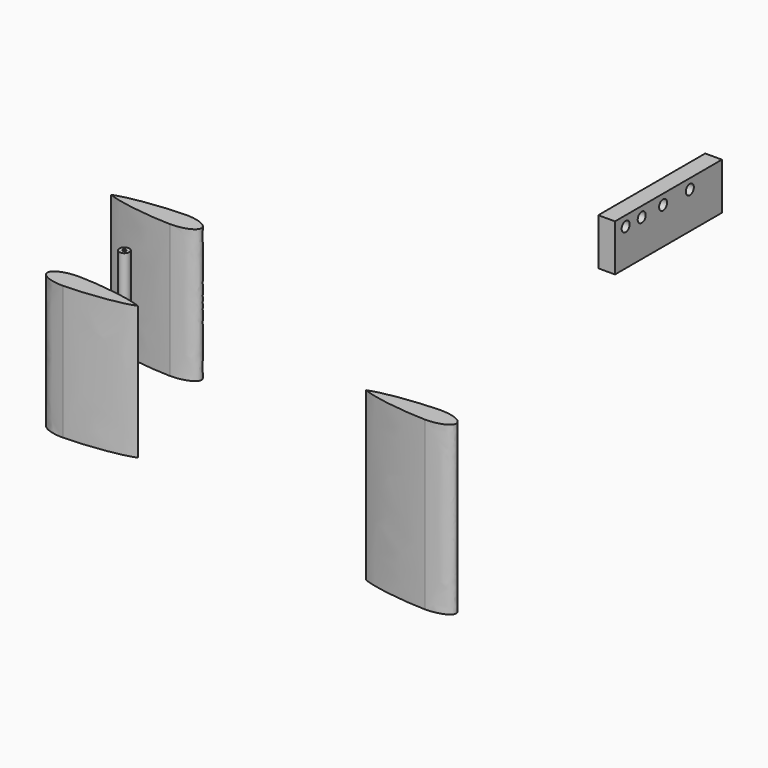
from build123d import *

# Parameters (mm, degrees)
F1_DEPTH = 250
F2_DEPTH = 200
F0_R     = 7.5
F0_R_2   = 2.5
F6_W     = 200
F6_H     = 70
F6_R     = 7.5
F7_DEPTH = 25


# Not quite as in the source:
# - ends of sketch curves that miss each other by under 0.0002 mm in the source are joined
# - the program builds the solid bodies; features that only make, move or delete a surface that nothing else refers to are left out


with BuildPart() as f1:
    # F0 (on Top) → F1 (new body)
    with BuildSketch(Plane.XY):
        with BuildLine():
            add(Edge.make_bspline(
                [(0, -15), (35.3319384158, -15), (35.3319384158, 0), (35.3319384158, 15), (0, 15)],
                knots=[1.5707963268, 1.5707963268, 1.5707963268, 3.1415926536, 3.1415926536, 4.7123889804, 4.7123889804, 4.7123889804], degree=2, weights=[1, 0.7071067812, 1, 0.7071067812, 1]))
            add(Edge.make_bspline(
                [(0, 15), (-16.2319140521, 15.0000000963), (-71.5773864947, 10.9885398261), (-100.0000014291, -1.909e-07)],
                knots=[0, 0, 0, 0, 101.1187435224, 101.1187435224, 101.1187435224, 101.1187435224], degree=3))
            add(Edge.make_bspline(
                [(0, -15), (-16.2319140521, -15.0000000963), (-71.5773864947, -10.9885398261), (-100.0000014291, -1.909e-07)],
                knots=[0, 0, 0, 0, 101.1187435224, 101.1187435224, 101.1187435224, 101.1187435224], degree=3))
        make_face()
    extrude(amount=-F1_DEPTH)


with BuildPart() as f2:
    # F0 (on Top) → F2 (new body)
    with BuildSketch(Plane.XY):
        with BuildLine():
            add(Edge.make_bspline(
                [(-301.4754507362, -114.9492457264), (-266.1435123205, -114.9492457264), (-266.1435123205, -99.9492457264), (-266.1435123205, -84.9492457264), (-301.4754507362, -84.9492457264)],
                knots=[1.5707963268, 1.5707963268, 1.5707963268, 3.1415926536, 3.1415926536, 4.7123889804, 4.7123889804, 4.7123889804], degree=2, weights=[1, 0.7071067812, 1, 0.7071067812, 1]))
            add(Edge.make_bspline(
                [(-301.4754507362, -84.9492457264), (-317.7073647883, -84.9492456301), (-373.0528372309, -88.9607059003), (-401.4754521653, -99.9492459173)],
                knots=[0, 0, 0, 0, 101.1187435224, 101.1187435224, 101.1187435224, 101.1187435224], degree=3))
            add(Edge.make_bspline(
                [(-301.4754507362, -114.9492457264), (-317.7073647883, -114.9492458228), (-373.0528372309, -110.9377855526), (-401.4754521653, -99.9492459173)],
                knots=[0, 0, 0, 0, 101.1187435224, 101.1187435224, 101.1187435224, 101.1187435224], degree=3))
        make_face()
    extrude(amount=F2_DEPTH)


with BuildPart() as f2b:
    # F0 (on Top) → F2, piece 2 (new body)
    with BuildSketch(Plane.XY):
        with BuildLine():
            add(Edge.make_bspline(
                [(-301.3535811887, -284.9492457264), (-285.1216671366, -284.9492456301), (-229.776194694, -288.9607059003), (-201.3535797596, -299.9492459173)],
                knots=[0, 0, 0, 0, 101.1187435224, 101.1187435224, 101.1187435224, 101.1187435224], degree=3))
            add(Edge.make_bspline(
                [(-301.3535811887, -284.9492457264), (-336.6855196045, -284.9492457264), (-336.6855196045, -299.9492457264), (-336.6855196045, -314.9492457264), (-301.3535811887, -314.9492457264)],
                knots=[4.7123889804, 4.7123889804, 4.7123889804, 6.2831853072, 6.2831853072, 7.853981634, 7.853981634, 7.853981634], degree=2, weights=[1, 0.7071067812, 1, 0.7071067812, 1]))
            add(Edge.make_bspline(
                [(-301.3535811887, -314.9492457264), (-285.1216671366, -314.9492458228), (-229.776194694, -310.9377855526), (-201.3535797596, -299.9492459173)],
                knots=[0, 0, 0, 0, 101.1187435224, 101.1187435224, 101.1187435224, 101.1187435224], degree=3))
        make_face()
    extrude(amount=F2_DEPTH)


with BuildPart() as f2c:
    # F0 (on Top) → F2, piece 3 (new body)
    with BuildSketch(Plane.XY):
        with Locations((-301.4754507362, -199.9492457264)):
            Circle(F0_R)
        with Locations((-301.4754507362, -199.9492457264)):
            Circle(F0_R_2, mode=Mode.SUBTRACT)
    extrude(amount=F2_DEPTH)


with BuildPart() as f7:
    # F6 (on Right) → F7 (new body)
    with BuildSketch(Plane.YZ):
        with Locations((409.4553355339, 102.2302365841)):
            Rectangle(F6_W, F6_H)
        with Locations((329.4553355339, 122.2302365841)):
            Circle(F6_R, mode=Mode.SUBTRACT)
        with Locations((359.4553355339, 122.2302365841)):
            Circle(F6_R, mode=Mode.SUBTRACT)
        with Locations((399.4553355339, 122.2302365841)):
            Circle(F6_R, mode=Mode.SUBTRACT)
        with Locations((449.4553355339, 122.2302365841)):
            Circle(F6_R, mode=Mode.SUBTRACT)
    extrude(amount=F7_DEPTH)


solid = Compound([f1.part, f2.part, f2b.part, f2c.part, f7.part])
